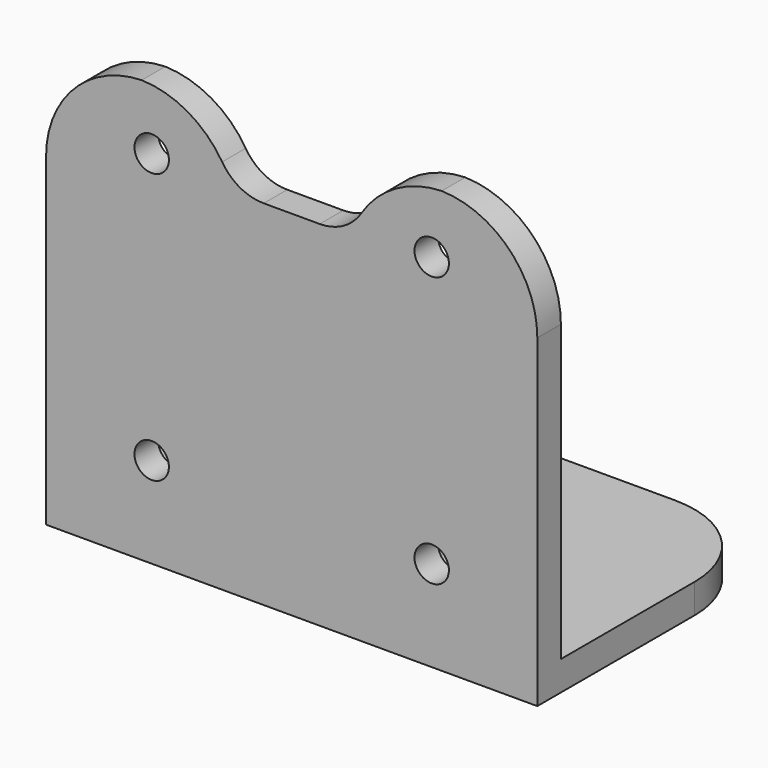
from build123d import *

# Parameters (mm, degrees)
F0_R        = 1.75
F1_DEPTH    = 3
F2_W        = 50
F2_H        = 3
F2_H_2      = 27
F2_R        = 1
F2_R_2      = 1.5
F3_DEPTH    = 3
F4_T1_DEPTH = 53
F4_T3_DEPTH = 53
F4_T5_DEPTH = 50.6969600708
F5_R        = 5


# Not quite as in the source:
# - a fillet or chamfer that OpenCascade refuses, or shapes differently, is made with other operations: its cross-section is extruded or revolved along the edge and cut away or added


with BuildPart() as f1:
    # F0 (on Front) → F1 (new body)
    with BuildSketch(Plane.XZ):
        Polygon((-6, 20), (-25, 20), (-25, -20), (25, -20), (25, 20), (6, 20), (6, 13), (-6, 13), align=None)
        with Locations((-14.25, -13.75)):
            Circle(F0_R, mode=Mode.SUBTRACT)
        with Locations((14.25, -13.75)):
            Circle(F0_R, mode=Mode.SUBTRACT)
        with Locations((-14.25, 13.75)):
            Circle(F0_R, mode=Mode.SUBTRACT)
        with Locations((14.25, 13.75)):
            Circle(F0_R, mode=Mode.SUBTRACT)
    extrude(amount=F1_DEPTH)

    # F2 (on face) → F3 (join)
    with BuildSketch(Plane(origin=(0, 0, -20), x_dir=(1, 0, 0), z_dir=(0, 0, -1))):
        with Locations((0, 1.5)):
            Rectangle(F2_W, F2_H)
        with Locations((0, -13.5)):
            Rectangle(F2_W, F2_H_2)
        with Locations((-8.5, -12.5)):
            Circle(F2_R, mode=Mode.SUBTRACT)
        with Locations((0, -22.5)):
            Circle(F2_R, mode=Mode.SUBTRACT)
        with Locations((0, -12.5)):
            Circle(F2_R_2, mode=Mode.SUBTRACT)
        with Locations((8.5, -12.5)):
            Circle(F2_R, mode=Mode.SUBTRACT)
    extrude(amount=F3_DEPTH)

    # F4: fillet of radius 10 on 6 edges, made by hand

    # F4_s2 → F4_t1 (cut)
    with BuildSketch(Plane.XY.offset(-48)):
        with BuildLine():
            ThreePointArc((25, 17), (22.0710678119, 24.0710678119), (15, 27))
            Line((15, 27), (25, 27))
            Line((25, 27), (25, 17))
        make_face()
        with BuildLine():
            ThreePointArc((-15, 27), (-22.0710678119, 24.0710678119), (-25, 17))
            Line((-25, 17), (-25, 27))
            Line((-25, 27), (-15, 27))
        make_face()
    extrude(amount=F4_T1_DEPTH, mode=Mode.SUBTRACT)

    # F4_s4 → F4_t3 (cut)
    with BuildSketch(Plane.XZ.offset(-25)):
        with BuildLine():
            ThreePointArc((-15, 20), (-22.0710678119, 17.0710678119), (-25, 10))
            Line((-25, 10), (-25, 20))
            Line((-25, 20), (-15, 20))
        make_face()
        with BuildLine():
            ThreePointArc((15, 20), (22.0710678119, 17.0710678119), (25, 10))
            Line((25, 10), (25, 20))
            Line((25, 20), (15, 20))
        make_face()
    extrude(amount=F4_T3_DEPTH, mode=Mode.SUBTRACT)

    # F4_s6 → F4_t5 (cut)
    with BuildSketch(Plane.XZ.offset(-23.8484800354)):
        with BuildLine():
            ThreePointArc((6, 13), (9.6233122311, 18.0622577483), (15.5393920142, 20))
            Line((15.5393920142, 20), (6, 20))
            Line((6, 20), (6, 13))
        make_face()
        with BuildLine():
            ThreePointArc((-15.5393920142, 20), (-9.6233122311, 18.0622577483), (-6, 13))
            Line((-6, 13), (-6, 20))
            Line((-6, 20), (-15.5393920142, 20))
        make_face()
    extrude(amount=F4_T5_DEPTH, mode=Mode.SUBTRACT)

    # F5
    f5_edges = [f1.edges().sort_by_distance(p)[0] for p in [
        (6, -1.5, 13),
        (-6, -1.5, 13),
    ]]
    fillet(f5_edges, radius=F5_R)


solid = f1.part
